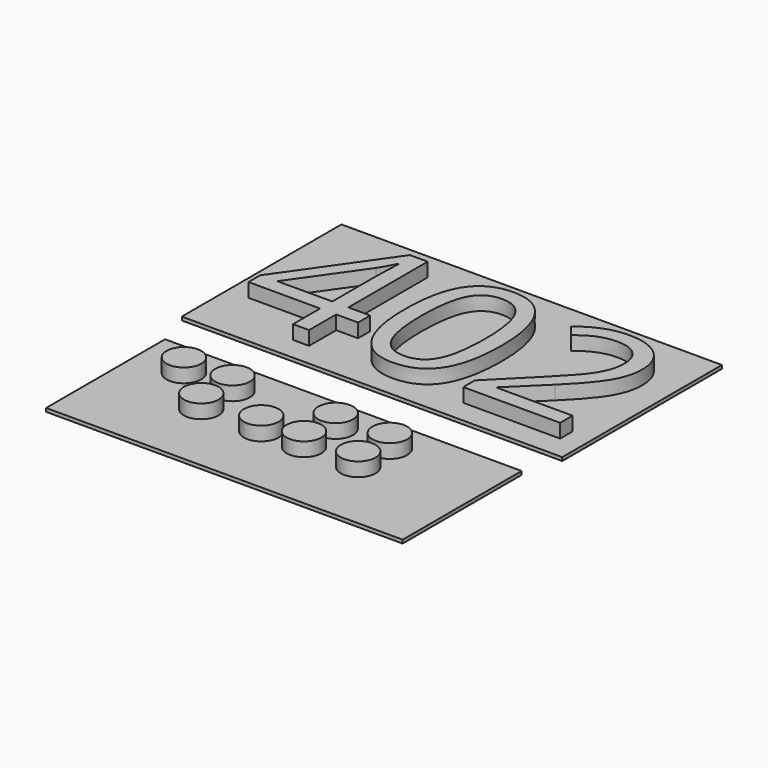
from build123d import *

# Parameters (mm, degrees)
F0_R         = 3.175
F0_TEXT_SIZE = 37.7791028263
F1_DEPTH     = 2.54
F2_W         = 65.2272
F2_H         = 27.2034
F2_W_2       = 69.6013405744
F2_H_2       = 36.5129876882
F3_DEPTH     = 0.635


# Not quite as in the source:
# - Text() gives the source's letters only with a copy of the font that has no kerning and outlines rounded to 1/6400 em; it was checked with that copy


with BuildPart() as f1:
    # F0 (on Top) → F1 (new body)
    with BuildSketch(Plane.XY):
        with Locations((-65.3789700321, 7.1374)):
            Circle(F0_R)
        with Locations((-27.7960782933, 7.239)):
            Circle(F0_R)
        with Locations((-37.7020782933, 7.239)):
            Circle(F0_R)
        with Locations((-27.7960782933, 0)):
            Circle(F0_R)
        with Locations((-37.7020782933, 0)):
            Circle(F0_R)
        with Locations((-45.5245375633, 0)):
            Circle(F0_R)
        with Locations((-56.4889700321, 7.1374)):
            Circle(F0_R)
        with Locations((-56.4980782933, 0)):
            Circle(F0_R)
        with Locations((-73.516080156, 24.8729400337)):
            Text('402', F0_TEXT_SIZE, font='Open Sans', text_align=(TextAlign.LEFT, TextAlign.BOTTOM))
    extrude(amount=F1_DEPTH)

    # F2 (on Top) → F3 (join)
    with BuildSketch(Plane.XY):
        with Locations((-41.402, 0.0127)):
            Rectangle(F2_W, F2_H)
        with Locations((-41.7344099034, 38.8409970328)):
            Rectangle(F2_W_2, F2_H_2)
    extrude(amount=-F3_DEPTH)


solid = f1.part
